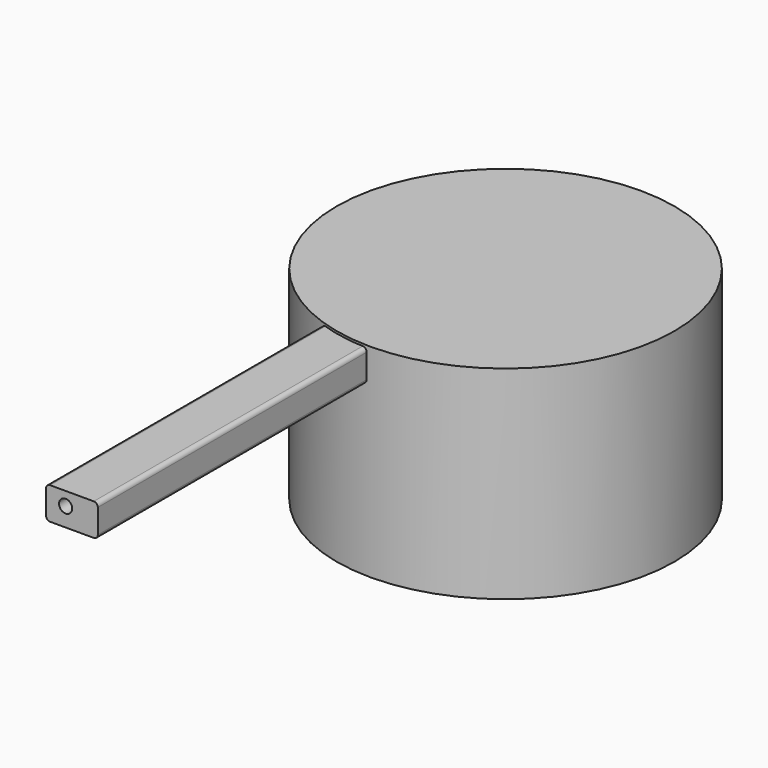
from build123d import *

# Parameters (mm, degrees)
F0_W     = 64.7000456229
F0_H     = 40.2752840891
F0_R     = 8.1996249531
F1_DEPTH = 533.4
F2_R     = 5.08
F3_R     = 211.3310828814
F4_DEPTH = 254


# Not quite as in the source:
# - a feature names something its author has since deleted; it is built from what else it names


with BuildPart() as f1:
    # F0 (on Front) → F1 (new body)
    with BuildSketch(Plane.XZ):
        with Locations((-37.2764277272, -22.9125614278)):
            Rectangle(F0_W, F0_H)
        with Locations((-45.1586656272, -19.5226017386)):
            Circle(F0_R, mode=Mode.SUBTRACT)
    extrude(amount=F1_DEPTH)

    # F2
    f2_edges = [f1.edges().sort_by_distance(p)[0] for p in [
        (-4.926405, -266.7, -2.774919),
        (-4.926405, -266.7, -43.050203),
        (-69.626451, -266.7, -2.774919),
        (-69.626451, -266.7, -43.050203),
    ]]
    fillet(f2_edges, radius=F2_R)


with BuildPart() as f4:
    # F3 (on Top) → F4 (new body)
    with BuildSketch(Plane.XY):
        with Locations((0, 97.9972705245)):
            Circle(F3_R)
    extrude(amount=-F4_DEPTH)


solid = Compound([f1.part, f4.part])
